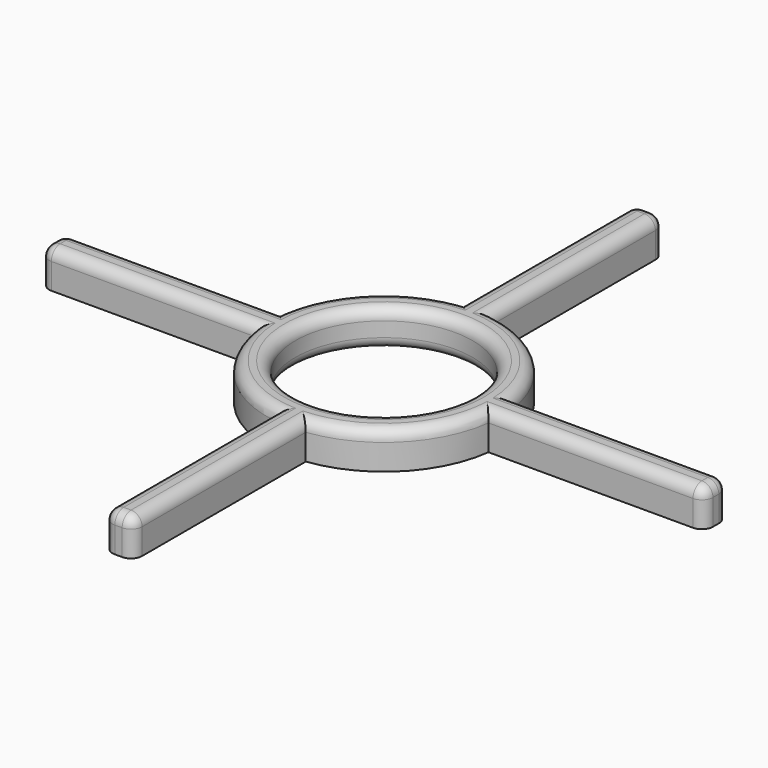
from build123d import *

# Parameters (mm, degrees)
F0_R         = 24
F1_DEPTH     = 10
F2_R         = 3
F3_T1_DEPTH  = 14.5
F3_S5_W      = 3
F3_S5_H      = 3
F3_T6_DEPTH  = 3
F3_S11_W     = 3
F3_S11_H     = 3
F3_T12_DEPTH = 3
F3_S17_W     = 3
F3_S17_H     = 3
F3_T18_DEPTH = 3
F3_S23_W     = 3
F3_S23_H     = 3
F3_T24_DEPTH = 3
F3_S29_W     = 3
F3_S29_H     = 3
F3_T30_DEPTH = 3
F3_S35_W     = 3
F3_S35_H     = 3
F3_T36_DEPTH = 3
F3_S41_W     = 3
F3_S41_H     = 3
F3_T42_DEPTH = 3
F3_S47_W     = 3
F3_S47_H     = 3
F3_T48_DEPTH = 3


# Not quite as in the source:
# - a fillet or chamfer that OpenCascade refuses, or shapes differently, is made with other operations: its cross-section is extruded or revolved along the edge and cut away or added


with BuildPart() as f1:
    # F0 (on Top) → F1 (new body)
    with BuildSketch(Plane.XY):
        with BuildLine():
            Line((31.5276851761, -4), (90, -4))
            Line((90, -4), (90, 4))
            Line((90, 4), (31.5276851761, 4))
            ThreePointArc((31.5276851761, 4), (22.4721486797, 22.4721486797), (4, 31.5276851761))
            Line((4, 31.5276851761), (4, 90))
            Line((4, 90), (-4, 90))
            Line((-4, 90), (-4, 31.5276851761))
            ThreePointArc((-4, 31.5276851761), (-22.4721486797, 22.4721486797), (-31.5276851761, 4))
            Line((-31.5276851761, 4), (-90, 4))
            Line((-90, 4), (-90, -4))
            Line((-90, -4), (-31.5276851761, -4))
            ThreePointArc((-31.5276851761, -4), (-22.4721486797, -22.4721486797), (-4, -31.5276851761))
            Line((-4, -31.5276851761), (-4, -90))
            Line((-4, -90), (4, -90))
            Line((4, -90), (4, -31.5276851761))
            ThreePointArc((4, -31.5276851761), (22.4721486797, -22.4721486797), (31.5276851761, -4))
        make_face()
        Circle(F0_R, mode=Mode.SUBTRACT)
    extrude(amount=F1_DEPTH)

    # F2
    f2_edges = [f1.edges().sort_by_distance(p)[0] for p in [
        (-22.472149, -22.472149, 10),
        (-4, -60.763843, 10),
        (0, -90, 10),
        (4, -60.763843, 10),
        (22.472149, -22.472149, 10),
        (60.763843, -4, 10),
        (90, 0, 10),
        (60.763843, 4, 10),
        (22.472149, 22.472149, 10),
        (4, 60.763843, 10),
        (0, 90, 10),
        (-4, 60.763843, 10),
        (-22.472149, 22.472149, 10),
        (-60.763843, 4, 10),
        (-90, 0, 10),
        (-60.763843, -4, 10),
        (-24, 0, 10),
    ]]
    fillet(f2_edges, radius=F2_R)

    # F3: fillet of radius 3 on 9 edges, made by hand

    # F3_s2 → F3_t1 (cut)
    with BuildSketch(Plane.XY.offset(-7.5)):
        with BuildLine():
            ThreePointArc((-87, -4), (-89.1213203436, -3.1213203436), (-90, -1))
            Line((-90, -1), (-90, -4))
            Line((-90, -4), (-87, -4))
        make_face()
        with BuildLine():
            ThreePointArc((-90, 1), (-89.1213203436, 3.1213203436), (-87, 4))
            Line((-87, 4), (-90, 4))
            Line((-90, 4), (-90, 1))
        make_face()
        with BuildLine():
            ThreePointArc((1, -90), (3.1213203436, -89.1213203436), (4, -87))
            Line((4, -87), (4, -90))
            Line((4, -90), (1, -90))
        make_face()
        with BuildLine():
            ThreePointArc((-4, -87), (-3.1213203436, -89.1213203436), (-1, -90))
            Line((-1, -90), (-4, -90))
            Line((-4, -90), (-4, -87))
        make_face()
        with BuildLine():
            ThreePointArc((87, -4), (89.1213203436, -3.1213203436), (90, -1))
            Line((90, -1), (90, -4))
            Line((90, -4), (87, -4))
        make_face()
        with BuildLine():
            ThreePointArc((90, 1), (89.1213203436, 3.1213203436), (87, 4))
            Line((87, 4), (90, 4))
            Line((90, 4), (90, 1))
        make_face()
        with BuildLine():
            ThreePointArc((4, 87), (3.1213203436, 89.1213203436), (1, 90))
            Line((1, 90), (4, 90))
            Line((4, 90), (4, 87))
        make_face()
        with BuildLine():
            ThreePointArc((-1, 90), (-3.1213203436, 89.1213203436), (-4, 87))
            Line((-4, 87), (-4, 90))
            Line((-4, 90), (-1, 90))
        make_face()
    extrude(amount=F3_T1_DEPTH, mode=Mode.SUBTRACT)


with BuildPart() as f3_tool4:
    # F3_s5 → F3_t6 (new body)
    with BuildSketch(Plane.XZ.offset(-87)):
        with Locations((-2.5, 8.5)):
            Rectangle(F3_S5_W, F3_S5_H)
    extrude(amount=-F3_T6_DEPTH)

    # F3_s7 → F3_t8 (revolve, cut)
    with BuildSketch(Plane(origin=(-1, 87, 7), x_dir=(0.7071067812, 0, -0.7071067812), z_dir=(0.7071067812, 0, 0.7071067812))):
        with BuildLine():
            ThreePointArc((0, -3), (3, 0), (0, 3))
            Line((0, 3), (0, -3))
        make_face()
    revolve(axis=Axis((-1, 87, 7), (0, 1, 0)), mode=Mode.SUBTRACT)


with BuildPart() as f1_1:
    add(f1.part)

    # F3_t3: cut F3_tool4
    add(f3_tool4.part, mode=Mode.SUBTRACT)


with BuildPart() as f3_tool10:
    # F3_s11 → F3_t12 (new body)
    with BuildSketch(Plane.YZ.offset(1)):
        with Locations((88.5, 8.5)):
            Rectangle(F3_S11_W, F3_S11_H)
    extrude(amount=F3_T12_DEPTH)

    # F3_s13 → F3_t14 (revolve, cut)
    with BuildSketch(Plane(origin=(1, 87, 7), x_dir=(0, -0.7071067812, -0.7071067812), z_dir=(0, -0.7071067812, 0.7071067812))):
        with BuildLine():
            ThreePointArc((0, -3), (3, 0), (0, 3))
            Line((0, 3), (0, -3))
        make_face()
    revolve(axis=Axis((1, 87, 7), (1, 0, 0)), mode=Mode.SUBTRACT)


with BuildPart() as f1_2:
    add(f1_1.part)

    # F3_t9: cut F3_tool10
    add(f3_tool10.part, mode=Mode.SUBTRACT)


with BuildPart() as f3_tool16:
    # F3_s17 → F3_t18 (new body)
    with BuildSketch(Plane.YZ.offset(87)):
        with Locations((2.5, 8.5)):
            Rectangle(F3_S17_W, F3_S17_H)
    extrude(amount=F3_T18_DEPTH)

    # F3_s19 → F3_t20 (revolve, cut)
    with BuildSketch(Plane(origin=(87, 1, 7), x_dir=(0, -0.7071067812, -0.7071067812), z_dir=(0, -0.7071067812, 0.7071067812))):
        with BuildLine():
            ThreePointArc((0, -3), (3, 0), (0, 3))
            Line((0, 3), (0, -3))
        make_face()
    revolve(axis=Axis((87, 1, 7), (1, 0, 0)), mode=Mode.SUBTRACT)


with BuildPart() as f1_3:
    add(f1_2.part)

    # F3_t15: cut F3_tool16
    add(f3_tool16.part, mode=Mode.SUBTRACT)


with BuildPart() as f3_tool22:
    # F3_s23 → F3_t24 (new body)
    with BuildSketch(Plane.XZ.offset(1)):
        with Locations((88.5, 8.5)):
            Rectangle(F3_S23_W, F3_S23_H)
    extrude(amount=F3_T24_DEPTH)

    # F3_s25 → F3_t26 (revolve, cut)
    with BuildSketch(Plane(origin=(87, -1, 7), x_dir=(-0.7071067812, 0, -0.7071067812), z_dir=(-0.7071067812, 0, 0.7071067812))):
        with BuildLine():
            ThreePointArc((0, -3), (3, 0), (0, 3))
            Line((0, 3), (0, -3))
        make_face()
    revolve(axis=Axis((87, -1, 7), (0, -1, 0)), mode=Mode.SUBTRACT)


with BuildPart() as f1_4:
    add(f1_3.part)

    # F3_t21: cut F3_tool22
    add(f3_tool22.part, mode=Mode.SUBTRACT)


with BuildPart() as f3_tool28:
    # F3_s29 → F3_t30 (new body)
    with BuildSketch(Plane.YZ.offset(-1)):
        with Locations((-88.5, 8.5)):
            Rectangle(F3_S29_W, F3_S29_H)
    extrude(amount=-F3_T30_DEPTH)

    # F3_s31 → F3_t32 (revolve, cut)
    with BuildSketch(Plane(origin=(-1, -87, 7), x_dir=(0, 0.7071067812, -0.7071067812), z_dir=(0, 0.7071067812, 0.7071067812))):
        with BuildLine():
            ThreePointArc((0, -3), (3, 0), (0, 3))
            Line((0, 3), (0, -3))
        make_face()
    revolve(axis=Axis((-1, -87, 7), (-1, 0, 0)), mode=Mode.SUBTRACT)


with BuildPart() as f1_5:
    add(f1_4.part)

    # F3_t27: cut F3_tool28
    add(f3_tool28.part, mode=Mode.SUBTRACT)


with BuildPart() as f3_tool34:
    # F3_s35 → F3_t36 (new body)
    with BuildSketch(Plane.XZ.offset(87)):
        with Locations((2.5, 8.5)):
            Rectangle(F3_S35_W, F3_S35_H)
    extrude(amount=F3_T36_DEPTH)

    # F3_s37 → F3_t38 (revolve, cut)
    with BuildSketch(Plane(origin=(1, -87, 7), x_dir=(-0.7071067812, 0, -0.7071067812), z_dir=(-0.7071067812, 0, 0.7071067812))):
        with BuildLine():
            ThreePointArc((0, -3), (3, 0), (0, 3))
            Line((0, 3), (0, -3))
        make_face()
    revolve(axis=Axis((1, -87, 7), (0, -1, 0)), mode=Mode.SUBTRACT)


with BuildPart() as f1_6:
    add(f1_5.part)

    # F3_t33: cut F3_tool34
    add(f3_tool34.part, mode=Mode.SUBTRACT)


with BuildPart() as f3_tool40:
    # F3_s41 → F3_t42 (new body)
    with BuildSketch(Plane.YZ.offset(-87)):
        with Locations((2.5, 8.5)):
            Rectangle(F3_S41_W, F3_S41_H)
    extrude(amount=-F3_T42_DEPTH)

    # F3_s43 → F3_t44 (revolve, cut)
    with BuildSketch(Plane(origin=(-87, 1, 7), x_dir=(0, -0.7071067812, -0.7071067812), z_dir=(0, 0.7071067812, -0.7071067812))):
        with BuildLine():
            ThreePointArc((0, -3), (3, 0), (0, 3))
            Line((0, 3), (0, -3))
        make_face()
    revolve(axis=Axis((-87, 1, 7), (-1, 0, 0)), mode=Mode.SUBTRACT)


with BuildPart() as f1_7:
    add(f1_6.part)

    # F3_t39: cut F3_tool40
    add(f3_tool40.part, mode=Mode.SUBTRACT)


with BuildPart() as f3_tool46:
    # F3_s47 → F3_t48 (new body)
    with BuildSketch(Plane.XZ.offset(1)):
        with Locations((-88.5, 8.5)):
            Rectangle(F3_S47_W, F3_S47_H)
    extrude(amount=F3_T48_DEPTH)

    # F3_s49 → F3_t50 (revolve, cut)
    with BuildSketch(Plane(origin=(-87, -1, 7), x_dir=(0.7071067812, 0, -0.7071067812), z_dir=(-0.7071067812, 0, -0.7071067812))):
        with BuildLine():
            ThreePointArc((0, -3), (3, 0), (0, 3))
            Line((0, 3), (0, -3))
        make_face()
    revolve(axis=Axis((-87, -1, 7), (0, -1, 0)), mode=Mode.SUBTRACT)


with BuildPart() as f1_8:
    add(f1_7.part)

    # F3_t45: cut F3_tool46
    add(f3_tool46.part, mode=Mode.SUBTRACT)

    # F3_s51 → F3_t52 (revolve, cut)
    with BuildSketch(Plane.XZ):
        with BuildLine():
            ThreePointArc((27, 0), (24.8786796564, 0.8786796564), (24, 3))
            Line((24, 3), (24, 0))
            Line((24, 0), (27, 0))
        make_face()
    revolve(axis=Axis((0, 0, 0), (0, 0, 1)), mode=Mode.SUBTRACT)


solid = f1_8.part
